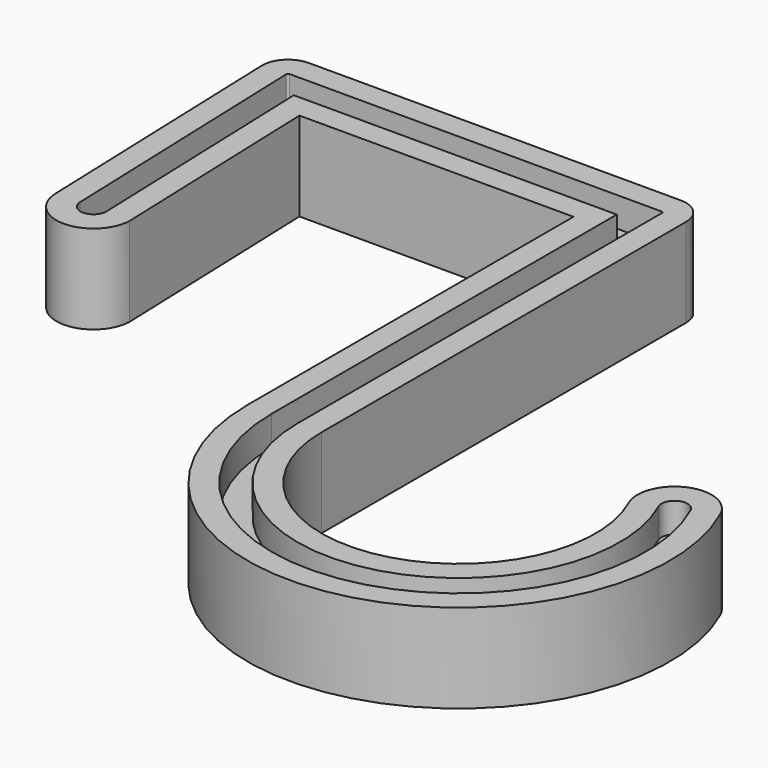
from build123d import *

# Parameters (mm, degrees)
F1_DEPTH = 12
F2_R     = 3.5
F4_DEPTH = 4
F6_DEPTH = 4


with BuildPart() as f1:
    # F0 (on Top) → F1 (new body)
    with BuildSketch(Plane.XY):
        with BuildLine():
            Line((10.9868871146, 38.4103373848), (-46.3684160233, 38.4103373848))
            Line((-46.3684160233, 38.4103373848), (-44.9722234273, -1.5713874258))
            ThreePointArc((-44.9722234273, -1.5713874258), (-39.9691757058, -6.4027744503), (-34.9661279843, -1.5713874258))
            Line((-34.9661279843, -1.5713874258), (-36.0131128854, 28.4103373848))
            Line((-36.0131128854, 28.4103373848), (0.9868871146, 28.4103373848))
            Line((0.9868871146, 28.4103373848), (0.9868871146, -26.5896626152))
            ThreePointArc((0.9868871146, -26.5896626152), (35.472835987, -54.4539482888), (55.4723899987, -14.8848072183))
            ThreePointArc((55.4723899987, -14.8848072183), (48.8600464406, -12.3794304662), (46.3546696885, -18.9917740242))
            ThreePointArc((46.3546696885, -18.9917740242), (33.3725030493, -44.6770059472), (10.9868871146, -26.5896626152))
            Line((10.9868871146, -26.5896626152), (10.9868871146, 38.4103373848))
        make_face()
    extrude(amount=F1_DEPTH)

    # F2
    f2_edges = [f1.edges().sort_by_distance(p)[0] for p in [
        (10.986887, 38.410337, 6),
        (-46.368416, 38.410337, 6),
    ]]
    fillet(f2_edges, radius=F2_R)

    # F3 (on face) → F4 (cut)
    with BuildSketch(Plane.XY.offset(12)):
        with BuildLine():
            Line((7.4868871146, 35.16033604), (-42.744059925, 35.16033604))
            ThreePointArc((-42.744059925, 35.16033604), (-42.9238939077, 35.0840010432), (-42.9939062878, 34.9016125575))
            Line((-42.9939062878, 34.9016125575), (-41.7242018955, -1.4579640146))
            ThreePointArc((-41.7242018955, -1.4579640146), (-40.0114090798, -3.1522651845), (-38.219126663, -1.5422839975))
            Line((-38.219126663, -1.5422839975), (-39.3785877977, 31.6603387296))
            Line((-39.3785877977, 31.6603387296), (4.2368884594, 31.6603387296))
            Line((4.2368884594, 31.6603387296), (4.2368884594, -26.5896626152))
            ThreePointArc((4.2368884594, -26.5896626152), (34.7902274998, -51.276440713), (52.5091296718, -16.2195719825))
            ThreePointArc((52.5091296718, -16.2195719825), (50.1948112049, -15.3426907931), (49.3179300155, -17.65700926))
            ThreePointArc((49.3179300155, -17.65700926), (34.0551115365, -47.854513523), (7.7368857699, -26.5896626152))
            Line((7.7368857699, -26.5896626152), (7.7368857699, 34.9103373848))
            ThreePointArc((7.7368857699, 34.9103373848), (7.663662859, 35.0871131292), (7.4868871146, 35.16033604))
        make_face()
    extrude(amount=-F4_DEPTH, mode=Mode.SUBTRACT)

    # F5 (on face) → F6 (cut)
    with BuildSketch(Plane(origin=(0, 0, 0), x_dir=(1, 0, 0), z_dir=(0, 0, -1))):
        with BuildLine():
            Line((-41.7242032033, 1.4579640602), (-42.9939075956, -34.9016125119))
            ThreePointArc((-42.9939075956, -34.9016125119), (-42.923894849, -35.0840019523), (-42.744059925, -35.1603373486))
            Line((-42.744059925, -35.1603373486), (7.4868871146, -35.1603373486))
            ThreePointArc((7.4868871146, -35.1603373486), (7.6636637843, -35.0871140545), (7.7368870784, -34.9103373848))
            Line((7.7368870784, -34.9103373848), (7.7368870784, 26.5896626152))
            ThreePointArc((7.7368870784, 26.5896626152), (34.0551112616, 47.8545122436), (49.3179288223, 17.6570097974))
            ThreePointArc((49.3179288223, 17.6570097974), (50.1948106674, 15.3426896), (52.5091308649, 16.2195714451))
            ThreePointArc((52.5091308649, 16.2195714451), (34.7902277746, 51.2764419924), (4.2368871508, 26.5896626152))
            Line((4.2368871508, 26.5896626152), (4.2368871508, -31.660337421))
            Line((4.2368871508, -31.660337421), (-39.3785864427, -31.660337421))
            Line((-39.3785864427, -31.660337421), (-38.2191253525, 1.5422840291))
            ThreePointArc((-38.2191253525, 1.5422840291), (-40.0114090726, 3.1522664936), (-41.7242032033, 1.4579640602))
        make_face()
    extrude(amount=-F6_DEPTH, mode=Mode.SUBTRACT)


solid = f1.part
